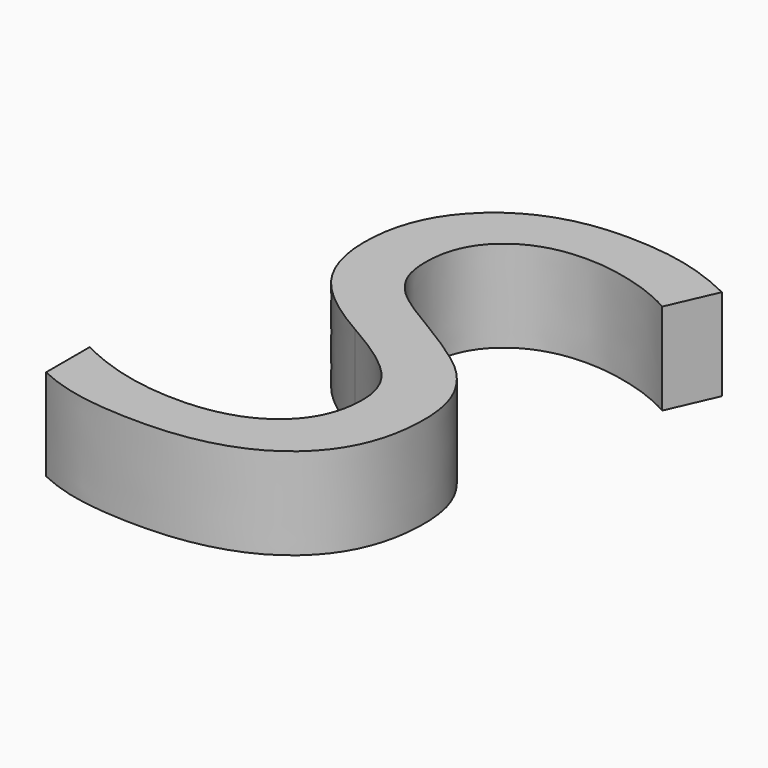
from build123d import *

# Parameters (mm, degrees)
F0_TEXT_SIZE = 78.9930578321
F1_DEPTH     = 11


# Not quite as in the source:
# - Text() gives the source's letters only with a copy of the font that has no kerning and outlines rounded to 1/6400 em; it was checked with that copy


with BuildPart() as f1:
    # F0 (on Top) → F1 (new body)
    with BuildSketch(Plane.XY):
        with Locations((-31.237501651, -28.4375008196)):
            Text('S', F0_TEXT_SIZE, font='Open Sans', font_style=FontStyle.ITALIC, text_align=(TextAlign.LEFT, TextAlign.BOTTOM))
    extrude(amount=F1_DEPTH)


solid = f1.part
